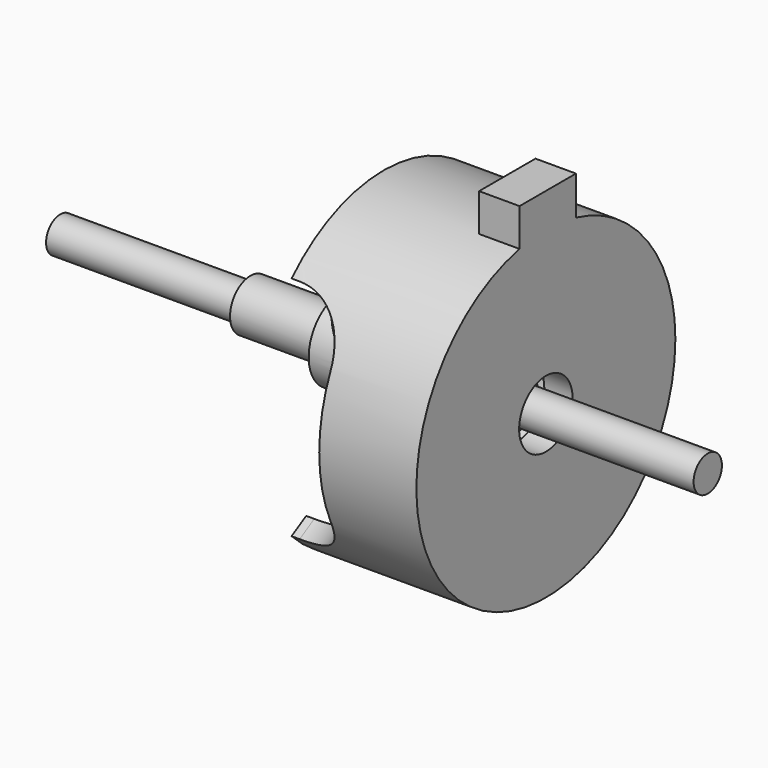
from build123d import *

# Parameters (mm, degrees)
F0_R      = 6.25
F1_DEPTH  = 33
F2_R      = 6.3
F3_DEPTH  = 33
F4_R      = 10.105326397
F5_DEPTH  = 10.5
F6_R      = 10.1267469355
F7_DEPTH  = 10.5
F8_R      = 7.0340005081
F9_DEPTH  = 16
F10_R     = 40
F10_R_2   = 35
F10_R_3   = 14
F11_DEPTH = 40
F12_DEPTH = 20
F13_DEPTH = 33
F15_DEPTH = 16
F16_R     = 14
F17_W     = 17.4193792045
F17_H     = 31.3548836857
F18_DEPTH = 10
F19_R     = 4.3759148518
F20_DEPTH = 80
F21_R     = 8.259826528
F22_DEPTH = 70


# Not quite as in the source:
# - a pattern or mirror of a feature is missing from the dataset's text; its kind, count and spacing are read off the source's solid


with BuildPart() as f1:
    # F0 (on Top) → F1 (new body, symmetric)
    with BuildSketch(Plane.XY):
        Circle(F0_R)
    extrude(amount=F1_DEPTH, both=True)

    # F2 (on Right) → F3 (join, symmetric)
    with BuildSketch(Plane.YZ):
        Circle(F2_R)
    extrude(amount=F3_DEPTH, both=True)

    # F4 (on Top) → F5 (join, symmetric)
    with BuildSketch(Plane.XY):
        Circle(F4_R)
    extrude(amount=F5_DEPTH, both=True)

    # F6 (on Right) → F7 (join, symmetric)
    with BuildSketch(Plane.YZ):
        Circle(F6_R)
    extrude(amount=F7_DEPTH, both=True)

    # F8 (on Front) → F9 (join)
    with BuildSketch(Plane.XZ):
        Circle(F8_R)
    extrude(amount=-F9_DEPTH)

    # F19 (on Right) → F20 (join, symmetric)
    with BuildSketch(Plane.YZ):
        Circle(F19_R)
    extrude(amount=F20_DEPTH, both=True)


with BuildPart() as f11:
    # F10 (on Right) → F11 (new body)
    with BuildSketch(Plane.YZ):
        Circle(F10_R)
        Circle(F10_R_2, mode=Mode.SUBTRACT)
        Circle(F10_R_2)
        Circle(F10_R_3, mode=Mode.SUBTRACT)
        Circle(F10_R_3)
    extrude(amount=F11_DEPTH)

    # F10 (on Right) → F12 (cut)
    with BuildSketch(Plane.YZ):
        Circle(F10_R_2)
        Circle(F10_R_3, mode=Mode.SUBTRACT)
    extrude(amount=F12_DEPTH, mode=Mode.SUBTRACT)

    # F10 (on Right) → F13 (cut)
    with BuildSketch(Plane.YZ):
        Circle(F10_R_3)
    extrude(amount=F13_DEPTH, mode=Mode.SUBTRACT)

    # F14 (on Right) → F15 (cut)
    with BuildSketch(Plane.YZ):
        with BuildLine():
            Line((-7.9614813968, 16.1435688114), (-29.4347208497, 28.5411493899))
            ThreePointArc((-29.4347208497, 28.5411493899), (-41, 0), (-29.4347208497, -28.5411493899))
            Line((-29.4347208497, -28.5411493899), (-7.9614813968, -16.1435688114))
            ThreePointArc((-7.9614813968, -16.1435688114), (-18, 0), (-7.9614813968, 16.1435688114))
        make_face()
    f15 = extrude(amount=F15_DEPTH, mode=Mode.SUBTRACT)

    # F15_copies: F15 across plane
    add(f15.mirror(Plane.ZX), mode=Mode.SUBTRACT)

    # F16
    f16_edges = [f11.edges().sort_by_distance(p)[0] for p in [
        (16, -26.294197, 26.727967),
        (16, -26.294197, -26.727967),
        (16, 26.294197, -26.727967),
        (16, 26.294197, 26.727967),
    ]]
    fillet(f16_edges, radius=F16_R)

    # F17 (on face) → F18 (join)
    with BuildSketch(Plane.YZ.offset(40)):
        with Locations((0.5806451663, 32.8064961359)):
            Rectangle(F17_W, F17_H)
    extrude(amount=-F18_DEPTH)

    # F21 (on Right) → F22 (cut)
    with BuildSketch(Plane.YZ):
        Circle(F21_R)
    extrude(amount=F22_DEPTH, mode=Mode.SUBTRACT)


solid = Compound([f1.part, f11.part])
